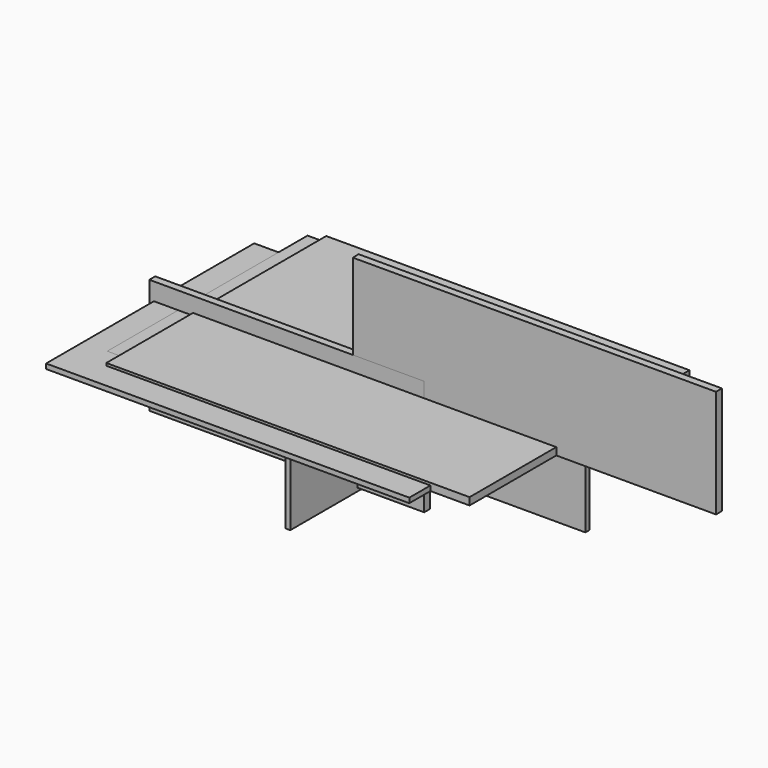
from build123d import *

# Parameters (mm, degrees)
F0_W      = 939.8
F0_H      = 279.4
F1_DEPTH  = 19.05
F2_W      = 939.8
F2_H      = 711.2
F3_DEPTH  = 19.05
F4_W      = 939.8
F4_H      = 673.1
F5_DEPTH  = 12.7
F6_W      = 711.2
F6_H      = 298.45
F7_DEPTH  = 19.05
F8_W      = 933.45
F8_H      = 203.2
F9_DEPTH  = 12.7
F10_W     = 622.3
F10_H     = 203.2
F11_DEPTH = 12.7
F12_W     = 933.45
F12_H     = 647.7
F13_DEPTH = 12.7


# Not quite as in the source:
# - a length typed as a fraction of an inch, garbled in the dataset ("3 / 203.2 mm" for 3/8 in), is restored


with BuildPart() as f1:
    # F0 (on Front) → F1 (new body)
    with BuildSketch(Plane.XZ):
        with Locations((469.9, 139.7)):
            Rectangle(F0_W, F0_H)
    extrude(amount=F1_DEPTH)


with BuildPart() as f3:
    # F2 (on Top) → F3 (new body)
    with BuildSketch(Plane.XY):
        with Locations((56.5968006849, 56.099815594)):
            Rectangle(F2_W, F2_H)
    extrude(amount=F3_DEPTH)


with BuildPart() as f5:
    # F4 (on Top) → F5 (new body)
    with BuildSketch(Plane.XY):
        with Locations((-44.6838438511, -31.1480367078)):
            Rectangle(F4_W, F4_H)
    extrude(amount=F5_DEPTH)


with BuildPart() as f7:
    # F6 (on Front) → F7 (new body)
    with BuildSketch(Plane.XZ):
        with Locations((-170.7684025168, -91.4403489557)):
            Rectangle(F6_W, F6_H)
    extrude(amount=F7_DEPTH)


with BuildPart() as f9:
    # F8 (on Front) → F9 (new body)
    with BuildSketch(Plane.XZ):
        with Locations((129.9587488174, -53.4627198363)):
            Rectangle(F8_W, F8_H)
    extrude(amount=F9_DEPTH)


with BuildPart() as f11:
    # F10 (on Right) → F11 (new body)
    with BuildSketch(Plane.YZ):
        with Locations((74.0094929934, -147.1401725494)):
            Rectangle(F10_W, F10_H)
    extrude(amount=F11_DEPTH)


with BuildPart() as f13:
    # F12 (on Top) → F13 (new body)
    with BuildSketch(Plane.XY):
        with Locations((15.0867402554, 75.3309479109)):
            Rectangle(F12_W, F12_H)
    extrude(amount=F13_DEPTH)


solid = Compound([f1.part, f3.part, f5.part, f7.part, f9.part, f11.part, f13.part])
